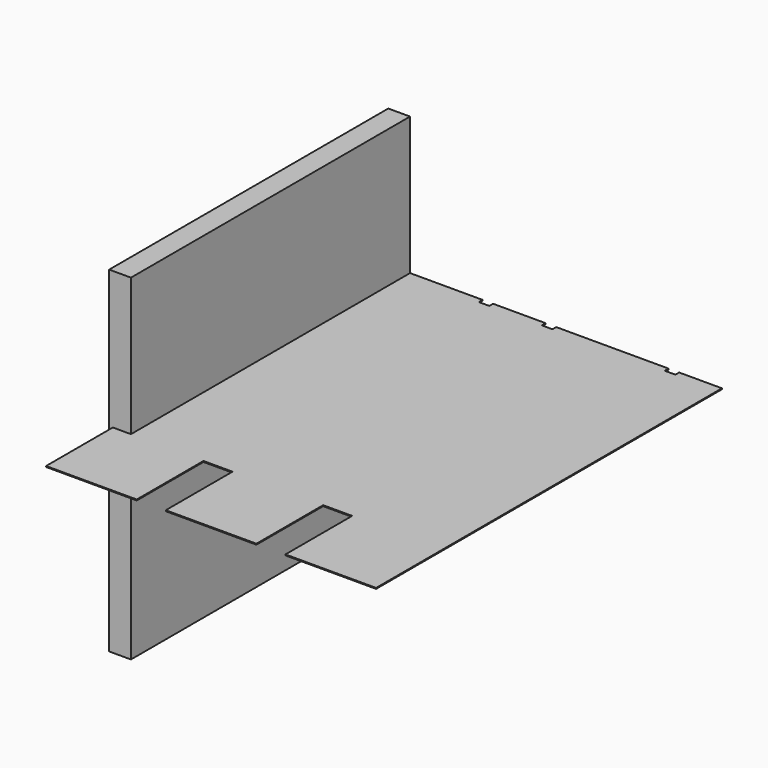
from build123d import *

# Parameters (mm, degrees)
F1_DEPTH = 25
F3_DEPTH = 5470
F4_DEPTH = 9270


# Not quite as in the source:
# - a feature names something its author has since deleted; it is built from what else it names


with BuildPart() as f1:
    # F0 (on Top) → F1 (new body)
    with BuildSketch(Plane.XY):
        Polygon((-3300, 0), (-2500, 0), (-2500, -2300), (0, -2300), (0, 0), (0, 9620), (-1180, 9620), (-1180, 9490), (-1470, 9490), (-1470, 9620), (-4570, 9620), (-4570, 9490), (-4860, 9490), (-4860, 9620), (-6310, 9620), (-6310, 9490), (-6600, 9490), (-6600, 9620), (-8600, 9620), (-8600, 0), (-9100, 0), (-9100, -2300), (-6600, -2300), (-6600, 0), (-5800, 0), (-5800, -2300), (-3300, -2300), align=None)
    extrude(amount=F1_DEPTH)



with BuildPart() as f3:
    # F2 (on face) → F3 (new body)
    with BuildSketch(Plane.XY.offset(25)):
        Polygon((-8600, 0), (-8600, 9620), (-9200, 9620), (-9200, 0), (-9100, 0), align=None)
    extrude(amount=-F3_DEPTH)


with BuildPart() as f1_1:
    add(f1.part)
    # F4 (add): a face of the model
    f4_faces = [f3.part.faces().sort_by_distance(p)[0] for p in [
        (-8900, 4810, -5445),
    ]]

    add(f3.part)  # F4 merges F3
    extrude(f4_faces, amount=-F4_DEPTH)


solid = f1_1.part
